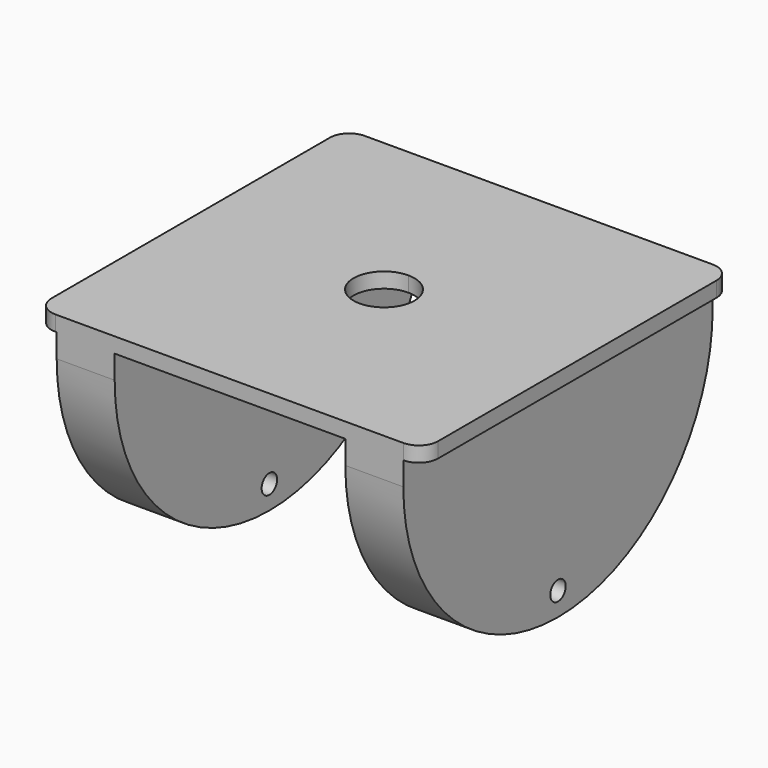
from build123d import *

# Parameters (mm, degrees)
F0_W     = 1.27
F0_H     = 25.4
F1_DEPTH = 1
F2_W     = 25.4
F2_H     = 14.24
F2_R     = 0.635
F2_H_2   = 1
F3_DEPTH = 3.81
F5_R     = 12.69999
F6_R     = 12.69999
F7_R     = 1.26999
F7_2_R   = 1.26999
F8_DEPTH = 0.0889


# Not quite as in the source:
# - a fillet or chamfer is up to 0.001 mm smaller than in the source, because OpenCascade refuses the exact size


with BuildPart() as f1:
    # F0 (on Top) → F1 (new body)
    with BuildSketch(Plane.XY):
        with Locations((-12.065, 0)):
            Rectangle(F0_W, F0_H)
    extrude(amount=F1_DEPTH)

    # F7 (radius 1.27 in the source; OpenCascade refuses exactly that, so slightly less here)
    f7_edges = [f1.edges().sort_by_distance(p)[0] for p in [
        (-12.7, -12.7, 0.5),
        (-12.7, 12.7, 0.5),
    ]]
    fillet(f7_edges, radius=F7_R)

    # F8 (add): a face of the model
    f8_faces = [f1.faces().sort_by_distance(p)[0] for p in [
        (-11.43, 0, 0.5),
    ]]


with BuildPart() as f1b:
    # F0 (on Top) → F1, piece 2 (new body)
    with BuildSketch(Plane.XY):
        with Locations((12.065, 0)):
            Rectangle(F0_W, F0_H)
    extrude(amount=F1_DEPTH)

    # F7#2 (radius 1.27 in the source; OpenCascade refuses exactly that, so slightly less here)
    f7_2_edges = [f1b.edges().sort_by_distance(p)[0] for p in [
        (12.7, -12.7, 0.5),
        (12.7, 12.7, 0.5),
    ]]
    fillet(f7_2_edges, radius=F7_2_R)


with BuildPart() as f1c:
    # F0 (on Top) → F1, piece 3 (new body)
    with BuildSketch(Plane.XY):
        with BuildLine():
            Line((0, -12.7), (7.62, -12.7))
            Line((7.62, -12.7), (7.62, 12.7))
            Line((7.62, 12.7), (0, 12.7))
            Line((0, 12.7), (0, 2))
            ThreePointArc((0, 2), (1.4142135624, 1.4142135624), (2, 0))
            ThreePointArc((2, 0), (1.4142135624, -1.4142135624), (0, -2))
            Line((0, -2), (0, -12.7))
        make_face()
        with BuildLine():
            Line((-7.62, -12.7), (0, -12.7))
            Line((0, -12.7), (0, -2))
            ThreePointArc((0, -2), (-2, 0), (0, 2))
            Line((0, 2), (0, 12.7))
            Line((0, 12.7), (-7.62, 12.7))
            Line((-7.62, 12.7), (-7.62, -12.7))
        make_face()
    extrude(amount=F1_DEPTH)


with BuildPart() as f3:
    # F2 (on face) → F3 (new body)
    with BuildSketch(Plane(origin=(11.43, 0, 0), x_dir=(0, -1, 0), z_dir=(-1, 0, 0))):
        with Locations((0, -7.12)):
            Rectangle(F2_W, F2_H)
        with Locations((0, -12.7)):
            Circle(F2_R, mode=Mode.SUBTRACT)
        with Locations((0, 0.5)):
            Rectangle(F2_W, F2_H_2)
    extrude(amount=F3_DEPTH)


with BuildPart() as f4_1:
    # F4: copy of F3
    add(f3.part.moved(Location((-18.961354, 0, 0))))

    # F6 (radius 12.7 in the source; OpenCascade refuses exactly that, so slightly less here)
    f6_edges = [f4_1.edges().sort_by_distance(p)[0] for p in [
        (-9.436354, -12.7, -14.24),
        (-9.436354, 12.7, -14.24),
    ]]
    fillet(f6_edges, radius=F6_R)


with BuildPart() as f3_1:
    add(f3.part)

    # F5 (radius 12.7 in the source; OpenCascade refuses exactly that, so slightly less here)
    f5_edges = [f3_1.edges().sort_by_distance(p)[0] for p in [
        (9.525, -12.7, -14.24),
        (9.525, 12.7, -14.24),
    ]]
    fillet(f5_edges, radius=F5_R)


with BuildPart() as f1_1:
    add(f1.part)

    add(f1b.part)  # F8 merges F1b

    add(f1c.part)  # F8 merges F1c

    add(f3_1.part)  # F8 merges F3

    add(f4_1.part)  # F8 merges F4_1
    extrude(f8_faces, amount=F8_DEPTH)


solid = f1_1.part
